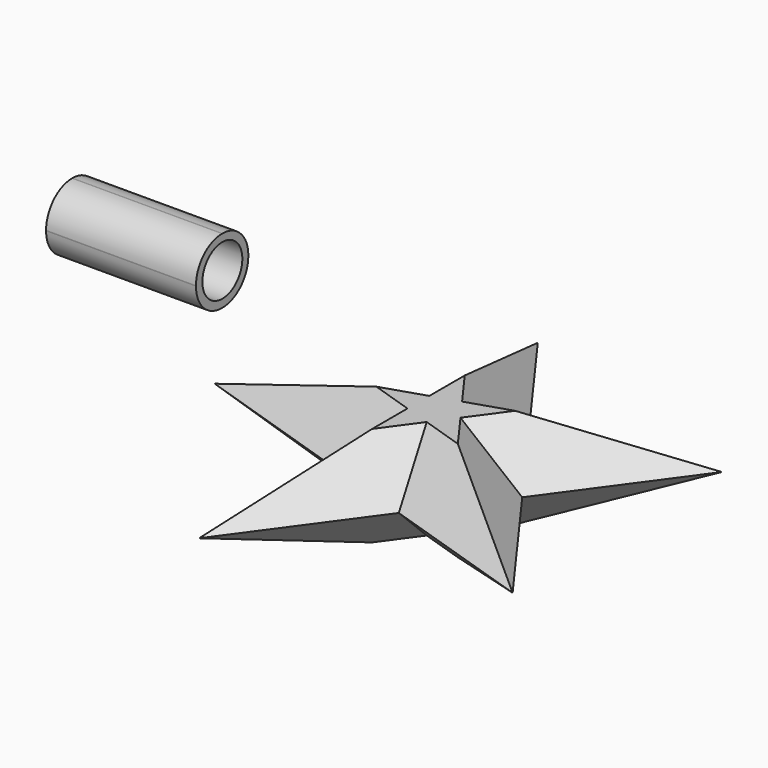
from build123d import *

# Parameters (mm, degrees)
F1_DEPTH      = 25.4
F2_T4_DEPTH   = 106.4188112086
F2_T9_DEPTH   = 106.4188112086
F2_T14_DEPTH  = 106.4188112086
F2_T19_DEPTH  = 106.4188112086
F2_T24_DEPTH  = 106.4188112086
F2_T29_DEPTH  = 106.4188112086
F2_T34_DEPTH  = 106.4188112086
F2_T39_DEPTH  = 106.4188112086
F2_T44_DEPTH  = 106.4188112086
F2_T49_DEPTH  = 106.4188112086
F2_T54_DEPTH  = 106.4188112086
F2_T59_DEPTH  = 106.4188112086
F2_T64_DEPTH  = 106.4188112086
F2_T69_DEPTH  = 106.4188112086
F2_T74_DEPTH  = 106.4188112086
F2_T79_DEPTH  = 106.4188112086
F2_T84_DEPTH  = 106.4188112086
F2_T89_DEPTH  = 106.4188112086
F2_T94_DEPTH  = 106.4188112086
F2_T99_DEPTH  = 106.4188112086
F2_T104_DEPTH = 106.4188112086
F2_T109_DEPTH = 106.4188112086
F2_T114_DEPTH = 106.4188112086
F2_T119_DEPTH = 106.4188112086
F2_T124_DEPTH = 106.4188112086
F2_T129_DEPTH = 106.4188112086
F2_T134_DEPTH = 106.4188112086
F2_T139_DEPTH = 106.4188112086
F2_T144_DEPTH = 106.4188112086
F2_T149_DEPTH = 106.4188112086
F2_T154_DEPTH = 106.4188112086
F2_T159_DEPTH = 106.4188112086
F2_T164_DEPTH = 106.4188112086
F2_T169_DEPTH = 106.4188112086
F2_T174_DEPTH = 106.4188112086
F2_T179_DEPTH = 106.4188112086
F2_T184_DEPTH = 106.4188112086
F2_T189_DEPTH = 106.4188112086
F2_T194_DEPTH = 106.4188112086
F2_T199_DEPTH = 106.4188112086
F2_T205_DEPTH = 106.4188112086
F2_T210_DEPTH = 106.4188112086
F2_T218_DEPTH = 106.4188112086
F2_T223_DEPTH = 106.4188112086
F2_T231_DEPTH = 106.4188112086
F2_T236_DEPTH = 106.4188112086
F2_T244_DEPTH = 106.4188112086
F2_T249_DEPTH = 106.4188112086
F2_T257_DEPTH = 106.4188112086
F2_T262_DEPTH = 106.4188112086
F2_T270_DEPTH = 106.4188112086
F2_T275_DEPTH = 106.4188112086
F2_T283_DEPTH = 106.4188112086
F2_T288_DEPTH = 106.4188112086
F2_T296_DEPTH = 106.4188112086
F2_T301_DEPTH = 106.4188112086
F2_T309_DEPTH = 106.4188112086
F2_T314_DEPTH = 106.4188112086
F2_T322_DEPTH = 106.4188112086
F2_T327_DEPTH = 106.4188112086
F3_W          = 38.1
F3_H          = 16.637
F4_DEPTH      = 16.637
F5_R          = 8.255
F6_R          = 6.35
F7_DEPTH      = 33.02


# Not quite as in the source:
# - a fillet or chamfer that OpenCascade refuses, or shapes differently, is made with other operations: its cross-section is extruded or revolved along the edge and cut away or added


with BuildPart() as f1:
    # F0 (on Top) → F1 (new body)
    with BuildSketch(Plane.XY):
        Polygon((45.763366046, 33.2490316571), (6.6767851239, 20.5490316571), (-17.48005039, 53.7980633142), (-17.48005039, 12.7), (-56.5666313121, 0), (-17.48005039, -12.7), (-17.48005039, -53.7980633142), (-5.401632633, -37.1735474857), (6.6767851239, -20.5490316571), (26.220075585, -26.8990316571), (45.763366046, -33.2490316571), (33.6849482891, -16.6245158286), (27.6457394106, -8.3122579143), (21.6065305321, 0), (27.6457394106, 8.3122579143), (33.6849482891, 16.6245158286), align=None)
    extrude(amount=F1_DEPTH)

    # F2: chamfer of 12.7 on 20 edges, made by hand


with BuildPart() as f2_tool2:
    # F2_s3 → F2_t4 (new body)
    with BuildSketch(Plane(origin=(82.2268601462, 26.7171264209, 0), x_dir=(0, 0, 1), z_dir=(-0.9510565163, -0.3090169944, 0))):
        Polygon((12.7, 17.48005039), (0, 4.78005039), (0, 17.48005039), align=None)
    extrude(amount=F2_T4_DEPTH)

    split(bisect_by=Plane(origin=(14.141657828, 10.2745158286, 0), x_dir=(0, 0, 1), z_dir=(0.8090169944, 0.5877852523, 0)), keep=Keep.TOP)


with BuildPart() as f1_1:
    add(f1.part)

    # F2_t1: cut F2_tool2
    add(f2_tool2.part, mode=Mode.SUBTRACT)


with BuildPart() as f2_tool7:
    # F2_s8 → F2_t9 (new body)
    with BuildSketch(Plane(origin=(82.2268601462, 26.7171264209, 0), x_dir=(0, 0, 1), z_dir=(-0.9510565163, -0.3090169944, 0))):
        Polygon((12.7, 17.48005039), (0, 4.78005039), (0, 17.48005039), align=None)
    extrude(amount=F2_T9_DEPTH)

    split(bisect_by=Plane.YZ.offset(-17.48005039), keep=Keep.BOTTOM)


with BuildPart() as f1_2:
    add(f1_1.part)

    # F2_t6: cut F2_tool7
    add(f2_tool7.part, mode=Mode.SUBTRACT)


with BuildPart() as f2_tool12:
    # F2_s13 → F2_t14 (new body)
    with BuildSketch(Plane(origin=(11.7324134364, -16.1482817373, 0), x_dir=(0, 0, 1), z_dir=(-0.5877852523, 0.8090169944, 0))):
        Polygon((12.7, 17.48005039), (0, 4.78005039), (0, 17.48005039), align=None)
    extrude(amount=F2_T14_DEPTH)

    split(bisect_by=Plane(origin=(14.141657828, -10.2745158286, 0), x_dir=(0, 0, 1), z_dir=(0.8090169944, -0.5877852523, 0)), keep=Keep.TOP)


with BuildPart() as f1_3:
    add(f1_2.part)

    # F2_t11: cut F2_tool12
    add(f2_tool12.part, mode=Mode.SUBTRACT)


with BuildPart() as f2_tool17:
    # F2_s18 → F2_t19 (new body)
    with BuildSketch(Plane(origin=(11.7324134364, -16.1482817373, 0), x_dir=(0, 0, 1), z_dir=(-0.5877852523, 0.8090169944, 0))):
        Polygon((12.7, 17.48005039), (0, 4.78005039), (0, 17.48005039), align=None)
    extrude(amount=F2_T19_DEPTH)

    split(bisect_by=Plane(origin=(-5.401632633, 16.6245158286, 0), x_dir=(0, 0, 1), z_dir=(-0.3090169944, 0.9510565163, 0)), keep=Keep.TOP)


with BuildPart() as f1_4:
    add(f1_3.part)

    # F2_t16: cut F2_tool17
    add(f2_tool17.part, mode=Mode.SUBTRACT)


with BuildPart() as f2_tool22:
    # F2_s23 → F2_t24 (new body)
    with BuildSketch(Plane.XZ.offset(-86.4584372614)):
        Polygon((-17.48005039, 12.7), (-4.78005039, 0), (-17.48005039, 0), align=None)
    extrude(amount=F2_T24_DEPTH)

    split(bisect_by=Plane(origin=(-5.401632633, 16.6245158286, 0), x_dir=(0, 0, 1), z_dir=(-0.3090169944, 0.9510565163, 0)), keep=Keep.TOP)


with BuildPart() as f1_5:
    add(f1_4.part)

    # F2_t21: cut F2_tool22
    add(f2_tool22.part, mode=Mode.SUBTRACT)


with BuildPart() as f2_tool27:
    # F2_s28 → F2_t29 (new body)
    with BuildSketch(Plane.XZ.offset(-86.4584372614)):
        Polygon((-17.48005039, 12.7), (-4.78005039, 0), (-17.48005039, 0), align=None)
    extrude(amount=F2_T29_DEPTH)

    split(bisect_by=Plane(origin=(-5.401632633, -16.6245158286, 0), x_dir=(0, 0, 1), z_dir=(-0.3090169944, -0.9510565163, 0)), keep=Keep.TOP)


with BuildPart() as f1_6:
    add(f1_5.part)

    # F2_t26: cut F2_tool27
    add(f2_tool27.part, mode=Mode.SUBTRACT)


with BuildPart() as f2_tool32:
    # F2_s33 → F2_t34 (new body)
    with BuildSketch(Plane(origin=(18.9834437101, 6.1680947638, 0), x_dir=(0, 0, 1), z_dir=(-0.9510565163, -0.3090169944, 0))):
        Polygon((12.7, 17.48005039), (0, 4.78005039), (0, 17.48005039), align=None)
    extrude(amount=F2_T34_DEPTH)

    split(bisect_by=Plane(origin=(14.141657828, 10.2745158286, 0), x_dir=(0, 0, 1), z_dir=(0.8090169944, 0.5877852523, 0)), keep=Keep.TOP)


with BuildPart() as f1_7:
    add(f1_6.part)

    # F2_t31: cut F2_tool32
    add(f2_tool32.part, mode=Mode.SUBTRACT)


with BuildPart() as f2_tool37:
    # F2_s38 → F2_t39 (new body)
    with BuildSketch(Plane(origin=(18.9834437101, 6.1680947638, 0), x_dir=(0, 0, 1), z_dir=(-0.9510565163, -0.3090169944, 0))):
        Polygon((12.7, 17.48005039), (0, 4.78005039), (0, 17.48005039), align=None)
    extrude(amount=F2_T39_DEPTH)

    split(bisect_by=Plane.YZ.offset(-17.48005039), keep=Keep.BOTTOM)


with BuildPart() as f1_8:
    add(f1_7.part)

    # F2_t36: cut F2_tool37
    add(f2_tool37.part, mode=Mode.SUBTRACT)


with BuildPart() as f2_tool42:
    # F2_s43 → F2_t44 (new body)
    with BuildSketch(Plane(origin=(-82.2268601462, 26.7171264209, 0), x_dir=(0, 0, 1), z_dir=(0.9510565163, -0.3090169944, 0))):
        Polygon((12.7, 17.48005039), (0, 4.78005039), (0, 17.48005039), align=None)
    extrude(amount=F2_T44_DEPTH)

    split(bisect_by=Plane.YZ.offset(-17.48005039), keep=Keep.BOTTOM)


with BuildPart() as f1_9:
    add(f1_8.part)

    # F2_t41: cut F2_tool42
    add(f2_tool42.part, mode=Mode.SUBTRACT)


with BuildPart() as f2_tool47:
    # F2_s48 → F2_t49 (new body)
    with BuildSketch(Plane(origin=(-82.2268601462, 26.7171264209, 0), x_dir=(0, 0, 1), z_dir=(0.9510565163, -0.3090169944, 0))):
        Polygon((12.7, 17.48005039), (0, 4.78005039), (0, 17.48005039), align=None)
    extrude(amount=F2_T49_DEPTH)

    split(bisect_by=Plane(origin=(14.141657828, -10.2745158286, 0), x_dir=(0, 0, 1), z_dir=(0.8090169944, -0.5877852523, 0)), keep=Keep.TOP)


with BuildPart() as f1_10:
    add(f1_9.part)

    # F2_t46: cut F2_tool47
    add(f2_tool47.part, mode=Mode.SUBTRACT)


with BuildPart() as f2_tool52:
    # F2_s53 → F2_t54 (new body)
    with BuildSketch(Plane.XZ.offset(-19.9603739472)):
        Polygon((-17.48005039, 12.7), (-4.78005039, 0), (-17.48005039, 0), align=None)
    extrude(amount=F2_T54_DEPTH)

    split(bisect_by=Plane(origin=(-5.401632633, 16.6245158286, 0), x_dir=(0, 0, 1), z_dir=(-0.3090169944, 0.9510565163, 0)), keep=Keep.TOP)


with BuildPart() as f1_11:
    add(f1_10.part)

    # F2_t51: cut F2_tool52
    add(f2_tool52.part, mode=Mode.SUBTRACT)


with BuildPart() as f2_tool57:
    # F2_s58 → F2_t59 (new body)
    with BuildSketch(Plane.XZ.offset(-19.9603739472)):
        Polygon((-17.48005039, 12.7), (-4.78005039, 0), (-17.48005039, 0), align=None)
    extrude(amount=F2_T59_DEPTH)

    split(bisect_by=Plane(origin=(-5.401632633, -16.6245158286, 0), x_dir=(0, 0, 1), z_dir=(-0.3090169944, -0.9510565163, 0)), keep=Keep.TOP)


with BuildPart() as f1_12:
    add(f1_11.part)

    # F2_t56: cut F2_tool57
    add(f2_tool57.part, mode=Mode.SUBTRACT)


with BuildPart() as f2_tool62:
    # F2_s63 → F2_t64 (new body)
    with BuildSketch(Plane(origin=(-50.8189943585, -69.9463450516, 0), x_dir=(0, 0, 1), z_dir=(0.5877852523, 0.8090169944, 0))):
        Polygon((12.7, 17.48005039), (0, 4.78005039), (0, 17.48005039), align=None)
    extrude(amount=F2_T64_DEPTH)

    split(bisect_by=Plane(origin=(-5.401632633, -16.6245158286, 0), x_dir=(0, 0, 1), z_dir=(-0.3090169944, -0.9510565163, 0)), keep=Keep.TOP)


with BuildPart() as f1_13:
    add(f1_12.part)

    # F2_t61: cut F2_tool62
    add(f2_tool62.part, mode=Mode.SUBTRACT)


with BuildPart() as f2_tool67:
    # F2_s68 → F2_t69 (new body)
    with BuildSketch(Plane(origin=(-50.8189943585, -69.9463450516, 0), x_dir=(0, 0, 1), z_dir=(0.5877852523, 0.8090169944, 0))):
        Polygon((12.7, 17.48005039), (0, 4.78005039), (0, 17.48005039), align=None)
    extrude(amount=F2_T69_DEPTH)

    split(bisect_by=Plane(origin=(14.141657828, 10.2745158286, 0), x_dir=(0, 0, 1), z_dir=(0.8090169944, 0.5877852523, 0)), keep=Keep.TOP)


with BuildPart() as f1_14:
    add(f1_13.part)

    # F2_t66: cut F2_tool67
    add(f2_tool67.part, mode=Mode.SUBTRACT)


with BuildPart() as f2_tool72:
    # F2_s73 → F2_t74 (new body)
    with BuildSketch(Plane(origin=(-18.9834437101, 6.1680947638, 0), x_dir=(0, 0, 1), z_dir=(0.9510565163, -0.3090169944, 0))):
        Polygon((12.7, 17.48005039), (0, 4.78005039), (0, 17.48005039), align=None)
    extrude(amount=F2_T74_DEPTH)

    split(bisect_by=Plane.YZ.offset(-17.48005039), keep=Keep.BOTTOM)


with BuildPart() as f1_15:
    add(f1_14.part)

    # F2_t71: cut F2_tool72
    add(f2_tool72.part, mode=Mode.SUBTRACT)


with BuildPart() as f2_tool77:
    # F2_s78 → F2_t79 (new body)
    with BuildSketch(Plane(origin=(-18.9834437101, 6.1680947638, 0), x_dir=(0, 0, 1), z_dir=(0.9510565163, -0.3090169944, 0))):
        Polygon((12.7, 17.48005039), (0, 4.78005039), (0, 17.48005039), align=None)
    extrude(amount=F2_T79_DEPTH)

    split(bisect_by=Plane(origin=(14.141657828, -10.2745158286, 0), x_dir=(0, 0, 1), z_dir=(0.8090169944, -0.5877852523, 0)), keep=Keep.TOP)


with BuildPart() as f1_16:
    add(f1_15.part)

    # F2_t76: cut F2_tool77
    add(f2_tool77.part, mode=Mode.SUBTRACT)


with BuildPart() as f2_tool82:
    # F2_s83 → F2_t84 (new body)
    with BuildSketch(Plane(origin=(50.8189943585, -69.9463450516, 0), x_dir=(0, 0, 1), z_dir=(-0.5877852523, 0.8090169944, 0))):
        Polygon((12.7, 17.48005039), (0, 4.78005039), (0, 17.48005039), align=None)
    extrude(amount=F2_T84_DEPTH)

    split(bisect_by=Plane(origin=(14.141657828, -10.2745158286, 0), x_dir=(0, 0, 1), z_dir=(0.8090169944, -0.5877852523, 0)), keep=Keep.TOP)


with BuildPart() as f1_17:
    add(f1_16.part)

    # F2_t81: cut F2_tool82
    add(f2_tool82.part, mode=Mode.SUBTRACT)


with BuildPart() as f2_tool87:
    # F2_s88 → F2_t89 (new body)
    with BuildSketch(Plane(origin=(50.8189943585, -69.9463450516, 0), x_dir=(0, 0, 1), z_dir=(-0.5877852523, 0.8090169944, 0))):
        Polygon((12.7, 17.48005039), (0, 4.78005039), (0, 17.48005039), align=None)
    extrude(amount=F2_T89_DEPTH)

    split(bisect_by=Plane(origin=(-5.401632633, 16.6245158286, 0), x_dir=(0, 0, 1), z_dir=(-0.3090169944, 0.9510565163, 0)), keep=Keep.TOP)


with BuildPart() as f1_18:
    add(f1_17.part)

    # F2_t86: cut F2_tool87
    add(f2_tool87.part, mode=Mode.SUBTRACT)


with BuildPart() as f2_tool92:
    # F2_s93 → F2_t94 (new body)
    with BuildSketch(Plane(origin=(-11.7324134364, -16.1482817373, 0), x_dir=(0, 0, 1), z_dir=(0.5877852523, 0.8090169944, 0))):
        Polygon((12.7, 17.48005039), (0, 4.78005039), (0, 17.48005039), align=None)
    extrude(amount=F2_T94_DEPTH)

    split(bisect_by=Plane(origin=(-5.401632633, -16.6245158286, 0), x_dir=(0, 0, 1), z_dir=(-0.3090169944, -0.9510565163, 0)), keep=Keep.TOP)


with BuildPart() as f1_19:
    add(f1_18.part)

    # F2_t91: cut F2_tool92
    add(f2_tool92.part, mode=Mode.SUBTRACT)


with BuildPart() as f2_tool97:
    # F2_s98 → F2_t99 (new body)
    with BuildSketch(Plane(origin=(-11.7324134364, -16.1482817373, 0), x_dir=(0, 0, 1), z_dir=(0.5877852523, 0.8090169944, 0))):
        Polygon((12.7, 17.48005039), (0, 4.78005039), (0, 17.48005039), align=None)
    extrude(amount=F2_T99_DEPTH)

    split(bisect_by=Plane(origin=(14.141657828, 10.2745158286, 0), x_dir=(0, 0, 1), z_dir=(0.8090169944, 0.5877852523, 0)), keep=Keep.TOP)


with BuildPart() as f1_20:
    add(f1_19.part)

    # F2_t96: cut F2_tool97
    add(f2_tool97.part, mode=Mode.SUBTRACT)


with BuildPart() as f2_tool102:
    # F2_s103 → F2_t104 (new body)
    with BuildSketch(Plane(origin=(50.8189943585, 69.9463450516, 0), x_dir=(0, 0, 1), z_dir=(-0.5877852523, -0.8090169944, 0))):
        Polygon((12.7, -17.48005039), (25.4, -4.78005039), (25.4, -17.48005039), align=None)
    extrude(amount=F2_T104_DEPTH)

    split(bisect_by=Plane(origin=(14.141657828, 10.2745158286, 0), x_dir=(0, 0, 1), z_dir=(0.8090169944, 0.5877852523, 0)), keep=Keep.TOP)


with BuildPart() as f1_21:
    add(f1_20.part)

    # F2_t101: cut F2_tool102
    add(f2_tool102.part, mode=Mode.SUBTRACT)


with BuildPart() as f2_tool107:
    # F2_s108 → F2_t109 (new body)
    with BuildSketch(Plane(origin=(50.8189943585, 69.9463450516, 0), x_dir=(0, 0, 1), z_dir=(-0.5877852523, -0.8090169944, 0))):
        Polygon((12.7, -17.48005039), (25.4, -4.78005039), (25.4, -17.48005039), align=None)
    extrude(amount=F2_T109_DEPTH)

    split(bisect_by=Plane(origin=(-5.401632633, -16.6245158286, 0), x_dir=(0, 0, 1), z_dir=(-0.3090169944, -0.9510565163, 0)), keep=Keep.TOP)


with BuildPart() as f1_22:
    add(f1_21.part)

    # F2_t106: cut F2_tool107
    add(f2_tool107.part, mode=Mode.SUBTRACT)


with BuildPart() as f2_tool112:
    # F2_s113 → F2_t114 (new body)
    with BuildSketch(Plane(origin=(82.2268601462, 26.7171264209, 0), x_dir=(0, 0, 1), z_dir=(-0.9510565163, -0.3090169944, 0))):
        Polygon((12.7, 17.48005039), (25.4, 4.78005039), (25.4, 17.48005039), align=None)
    extrude(amount=F2_T114_DEPTH)

    split(bisect_by=Plane(origin=(14.141657828, 10.2745158286, 0), x_dir=(0, 0, 1), z_dir=(0.8090169944, 0.5877852523, 0)), keep=Keep.TOP)


with BuildPart() as f1_23:
    add(f1_22.part)

    # F2_t111: cut F2_tool112
    add(f2_tool112.part, mode=Mode.SUBTRACT)


with BuildPart() as f2_tool117:
    # F2_s118 → F2_t119 (new body)
    with BuildSketch(Plane(origin=(82.2268601462, 26.7171264209, 0), x_dir=(0, 0, 1), z_dir=(-0.9510565163, -0.3090169944, 0))):
        Polygon((12.7, 17.48005039), (25.4, 4.78005039), (25.4, 17.48005039), align=None)
    extrude(amount=F2_T119_DEPTH)

    split(bisect_by=Plane.YZ.offset(-17.48005039), keep=Keep.BOTTOM)


with BuildPart() as f1_24:
    add(f1_23.part)

    # F2_t116: cut F2_tool117
    add(f2_tool117.part, mode=Mode.SUBTRACT)


with BuildPart() as f2_tool122:
    # F2_s123 → F2_t124 (new body)
    with BuildSketch(Plane(origin=(11.7324134364, -16.1482817373, 0), x_dir=(0, 0, 1), z_dir=(-0.5877852523, 0.8090169944, 0))):
        Polygon((12.7, 17.48005039), (25.4, 4.78005039), (25.4, 17.48005039), align=None)
    extrude(amount=F2_T124_DEPTH)

    split(bisect_by=Plane(origin=(14.141657828, -10.2745158286, 0), x_dir=(0, 0, 1), z_dir=(0.8090169944, -0.5877852523, 0)), keep=Keep.TOP)


with BuildPart() as f1_25:
    add(f1_24.part)

    # F2_t121: cut F2_tool122
    add(f2_tool122.part, mode=Mode.SUBTRACT)


with BuildPart() as f2_tool127:
    # F2_s128 → F2_t129 (new body)
    with BuildSketch(Plane(origin=(11.7324134364, -16.1482817373, 0), x_dir=(0, 0, 1), z_dir=(-0.5877852523, 0.8090169944, 0))):
        Polygon((12.7, 17.48005039), (25.4, 4.78005039), (25.4, 17.48005039), align=None)
    extrude(amount=F2_T129_DEPTH)

    split(bisect_by=Plane(origin=(-5.401632633, 16.6245158286, 0), x_dir=(0, 0, 1), z_dir=(-0.3090169944, 0.9510565163, 0)), keep=Keep.TOP)


with BuildPart() as f1_26:
    add(f1_25.part)

    # F2_t126: cut F2_tool127
    add(f2_tool127.part, mode=Mode.SUBTRACT)


with BuildPart() as f2_tool132:
    # F2_s133 → F2_t134 (new body)
    with BuildSketch(Plane.XZ.offset(-86.4584372614)):
        Polygon((-17.48005039, 12.7), (-4.78005039, 25.4), (-17.48005039, 25.4), align=None)
    extrude(amount=F2_T134_DEPTH)

    split(bisect_by=Plane(origin=(-5.401632633, 16.6245158286, 0), x_dir=(0, 0, 1), z_dir=(-0.3090169944, 0.9510565163, 0)), keep=Keep.TOP)


with BuildPart() as f1_27:
    add(f1_26.part)

    # F2_t131: cut F2_tool132
    add(f2_tool132.part, mode=Mode.SUBTRACT)


with BuildPart() as f2_tool137:
    # F2_s138 → F2_t139 (new body)
    with BuildSketch(Plane.XZ.offset(-86.4584372614)):
        Polygon((-17.48005039, 12.7), (-4.78005039, 25.4), (-17.48005039, 25.4), align=None)
    extrude(amount=F2_T139_DEPTH)

    split(bisect_by=Plane(origin=(-5.401632633, -16.6245158286, 0), x_dir=(0, 0, 1), z_dir=(-0.3090169944, -0.9510565163, 0)), keep=Keep.TOP)


with BuildPart() as f1_28:
    add(f1_27.part)

    # F2_t136: cut F2_tool137
    add(f2_tool137.part, mode=Mode.SUBTRACT)


with BuildPart() as f2_tool142:
    # F2_s143 → F2_t144 (new body)
    with BuildSketch(Plane(origin=(18.9834437101, 6.1680947638, 0), x_dir=(0, 0, 1), z_dir=(-0.9510565163, -0.3090169944, 0))):
        Polygon((12.7, 17.48005039), (25.4, 4.78005039), (25.4, 17.48005039), align=None)
    extrude(amount=F2_T144_DEPTH)

    split(bisect_by=Plane(origin=(14.141657828, 10.2745158286, 0), x_dir=(0, 0, 1), z_dir=(0.8090169944, 0.5877852523, 0)), keep=Keep.TOP)


with BuildPart() as f1_29:
    add(f1_28.part)

    # F2_t141: cut F2_tool142
    add(f2_tool142.part, mode=Mode.SUBTRACT)


with BuildPart() as f2_tool147:
    # F2_s148 → F2_t149 (new body)
    with BuildSketch(Plane(origin=(18.9834437101, 6.1680947638, 0), x_dir=(0, 0, 1), z_dir=(-0.9510565163, -0.3090169944, 0))):
        Polygon((12.7, 17.48005039), (25.4, 4.78005039), (25.4, 17.48005039), align=None)
    extrude(amount=F2_T149_DEPTH)

    split(bisect_by=Plane.YZ.offset(-17.48005039), keep=Keep.BOTTOM)


with BuildPart() as f1_30:
    add(f1_29.part)

    # F2_t146: cut F2_tool147
    add(f2_tool147.part, mode=Mode.SUBTRACT)


with BuildPart() as f2_tool152:
    # F2_s153 → F2_t154 (new body)
    with BuildSketch(Plane(origin=(-82.2268601462, 26.7171264209, 0), x_dir=(0, 0, 1), z_dir=(0.9510565163, -0.3090169944, 0))):
        Polygon((12.7, 17.48005039), (25.4, 4.78005039), (25.4, 17.48005039), align=None)
    extrude(amount=F2_T154_DEPTH)

    split(bisect_by=Plane.YZ.offset(-17.48005039), keep=Keep.BOTTOM)


with BuildPart() as f1_31:
    add(f1_30.part)

    # F2_t151: cut F2_tool152
    add(f2_tool152.part, mode=Mode.SUBTRACT)


with BuildPart() as f2_tool157:
    # F2_s158 → F2_t159 (new body)
    with BuildSketch(Plane(origin=(-82.2268601462, 26.7171264209, 0), x_dir=(0, 0, 1), z_dir=(0.9510565163, -0.3090169944, 0))):
        Polygon((12.7, 17.48005039), (25.4, 4.78005039), (25.4, 17.48005039), align=None)
    extrude(amount=F2_T159_DEPTH)

    split(bisect_by=Plane(origin=(14.141657828, -10.2745158286, 0), x_dir=(0, 0, 1), z_dir=(0.8090169944, -0.5877852523, 0)), keep=Keep.TOP)


with BuildPart() as f1_32:
    add(f1_31.part)

    # F2_t156: cut F2_tool157
    add(f2_tool157.part, mode=Mode.SUBTRACT)


with BuildPart() as f2_tool162:
    # F2_s163 → F2_t164 (new body)
    with BuildSketch(Plane.XZ.offset(-19.9603739472)):
        Polygon((-17.48005039, 12.7), (-4.78005039, 25.4), (-17.48005039, 25.4), align=None)
    extrude(amount=F2_T164_DEPTH)

    split(bisect_by=Plane(origin=(-5.401632633, 16.6245158286, 0), x_dir=(0, 0, 1), z_dir=(-0.3090169944, 0.9510565163, 0)), keep=Keep.TOP)


with BuildPart() as f1_33:
    add(f1_32.part)

    # F2_t161: cut F2_tool162
    add(f2_tool162.part, mode=Mode.SUBTRACT)


with BuildPart() as f2_tool167:
    # F2_s168 → F2_t169 (new body)
    with BuildSketch(Plane.XZ.offset(-19.9603739472)):
        Polygon((-17.48005039, 12.7), (-4.78005039, 25.4), (-17.48005039, 25.4), align=None)
    extrude(amount=F2_T169_DEPTH)

    split(bisect_by=Plane(origin=(-5.401632633, -16.6245158286, 0), x_dir=(0, 0, 1), z_dir=(-0.3090169944, -0.9510565163, 0)), keep=Keep.TOP)


with BuildPart() as f1_34:
    add(f1_33.part)

    # F2_t166: cut F2_tool167
    add(f2_tool167.part, mode=Mode.SUBTRACT)


with BuildPart() as f2_tool172:
    # F2_s173 → F2_t174 (new body)
    with BuildSketch(Plane(origin=(11.7324134364, 16.1482817373, 0), x_dir=(0, 0, 1), z_dir=(-0.5877852523, -0.8090169944, 0))):
        Polygon((12.7, -17.48005039), (25.4, -4.78005039), (25.4, -17.48005039), align=None)
    extrude(amount=F2_T174_DEPTH)

    split(bisect_by=Plane(origin=(14.141657828, 10.2745158286, 0), x_dir=(0, 0, 1), z_dir=(0.8090169944, 0.5877852523, 0)), keep=Keep.TOP)


with BuildPart() as f1_35:
    add(f1_34.part)

    # F2_t171: cut F2_tool172
    add(f2_tool172.part, mode=Mode.SUBTRACT)


with BuildPart() as f2_tool177:
    # F2_s178 → F2_t179 (new body)
    with BuildSketch(Plane(origin=(11.7324134364, 16.1482817373, 0), x_dir=(0, 0, 1), z_dir=(-0.5877852523, -0.8090169944, 0))):
        Polygon((12.7, -17.48005039), (25.4, -4.78005039), (25.4, -17.48005039), align=None)
    extrude(amount=F2_T179_DEPTH)

    split(bisect_by=Plane(origin=(-5.401632633, -16.6245158286, 0), x_dir=(0, 0, 1), z_dir=(-0.3090169944, -0.9510565163, 0)), keep=Keep.TOP)


with BuildPart() as f1_36:
    add(f1_35.part)

    # F2_t176: cut F2_tool177
    add(f2_tool177.part, mode=Mode.SUBTRACT)


with BuildPart() as f2_tool182:
    # F2_s183 → F2_t184 (new body)
    with BuildSketch(Plane(origin=(82.2268601462, -26.7171264209, 0), x_dir=(0, 0, 1), z_dir=(-0.9510565163, 0.3090169944, 0))):
        Polygon((12.7, -17.48005039), (25.4, -4.78005039), (25.4, -17.48005039), align=None)
    extrude(amount=F2_T184_DEPTH)

    split(bisect_by=Plane(origin=(14.141657828, -10.2745158286, 0), x_dir=(0, 0, 1), z_dir=(0.8090169944, -0.5877852523, 0)), keep=Keep.TOP)


with BuildPart() as f1_37:
    add(f1_36.part)

    # F2_t181: cut F2_tool182
    add(f2_tool182.part, mode=Mode.SUBTRACT)


with BuildPart() as f2_tool187:
    # F2_s188 → F2_t189 (new body)
    with BuildSketch(Plane(origin=(82.2268601462, -26.7171264209, 0), x_dir=(0, 0, 1), z_dir=(-0.9510565163, 0.3090169944, 0))):
        Polygon((12.7, -17.48005039), (25.4, -4.78005039), (25.4, -17.48005039), align=None)
    extrude(amount=F2_T189_DEPTH)

    split(bisect_by=Plane.YZ.offset(-17.48005039), keep=Keep.BOTTOM)


with BuildPart() as f1_38:
    add(f1_37.part)

    # F2_t186: cut F2_tool187
    add(f2_tool187.part, mode=Mode.SUBTRACT)


with BuildPart() as f2_tool192:
    # F2_s193 → F2_t194 (new body)
    with BuildSketch(Plane(origin=(-11.7324134364, 16.1482817373, 0), x_dir=(0, 0, 1), z_dir=(0.5877852523, -0.8090169944, 0))):
        Polygon((25.4, -4.78005039), (12.7, -17.48005039), (25.4, -17.48005039), align=None)
    extrude(amount=F2_T194_DEPTH)

    split(bisect_by=Plane(origin=(-5.401632633, 16.6245158286, 0), x_dir=(0, 0, 1), z_dir=(-0.3090169944, 0.9510565163, 0)), keep=Keep.TOP)


with BuildPart() as f1_39:
    add(f1_38.part)

    # F2_t191: cut F2_tool192
    add(f2_tool192.part, mode=Mode.SUBTRACT)


with BuildPart() as f2_tool197:
    # F2_s198 → F2_t199 (new body)
    with BuildSketch(Plane(origin=(-11.7324134364, 16.1482817373, 0), x_dir=(0, 0, 1), z_dir=(0.5877852523, -0.8090169944, 0))):
        Polygon((25.4, -4.78005039), (12.7, -17.48005039), (25.4, -17.48005039), align=None)
    extrude(amount=F2_T199_DEPTH)

    split(bisect_by=Plane(origin=(14.141657828, -10.2745158286, 0), x_dir=(0, 0, 1), z_dir=(0.8090169944, -0.5877852523, 0)), keep=Keep.TOP)


with BuildPart() as f1_40:
    add(f1_39.part)

    # F2_t196: cut F2_tool197
    add(f2_tool197.part, mode=Mode.SUBTRACT)


with BuildPart() as f2_tool203:
    # F2_s204 → F2_t205 (new body)
    with BuildSketch(Plane(origin=(82.2268601462, 26.7171264209, 0), x_dir=(0, 0, 1), z_dir=(-0.9510565163, -0.3090169944, 0))):
        Polygon((12.7, 17.48005039), (0, 4.78005039), (0, 17.48005039), align=None)
    extrude(amount=F2_T205_DEPTH)

    split(bisect_by=Plane(origin=(14.141657828, 10.2745158286, 0), x_dir=(0, 0, 1), z_dir=(-0.8090169944, -0.5877852523, 0)), keep=Keep.TOP)

    split(bisect_by=Plane.YZ.offset(-17.48005039), keep=Keep.TOP)


with BuildPart() as f2_tool208:
    # F2_s209 → F2_t210 (new body)
    with BuildSketch(Plane(origin=(11.7324134364, -16.1482817373, 0), x_dir=(0, 0, 1), z_dir=(-0.5877852523, 0.8090169944, 0))):
        Polygon((12.7, 17.48005039), (0, 4.78005039), (0, 17.48005039), align=None)
    extrude(amount=F2_T210_DEPTH)

    split(bisect_by=Plane(origin=(14.141657828, -10.2745158286, 0), x_dir=(0, 0, 1), z_dir=(-0.8090169944, 0.5877852523, 0)), keep=Keep.TOP)

    split(bisect_by=Plane(origin=(-5.401632633, 16.6245158286, 0), x_dir=(0, 0, 1), z_dir=(0.3090169944, -0.9510565163, 0)), keep=Keep.TOP)


with BuildPart() as f2_tool203_1:
    add(f2_tool203.part)

    # F2_t213: intersect F2_tool208
    add(f2_tool208.part, mode=Mode.INTERSECT)


with BuildPart() as f1_41:
    add(f1_40.part)

    # F2_t201: cut F2_tool203
    add(f2_tool203_1.part, mode=Mode.SUBTRACT)


with BuildPart() as f2_tool216:
    # F2_s217 → F2_t218 (new body)
    with BuildSketch(Plane.XZ.offset(-86.4584372614)):
        Polygon((-17.48005039, 12.7), (-4.78005039, 0), (-17.48005039, 0), align=None)
    extrude(amount=F2_T218_DEPTH)

    split(bisect_by=Plane(origin=(-5.401632633, 16.6245158286, 0), x_dir=(0, 0, 1), z_dir=(0.3090169944, -0.9510565163, 0)), keep=Keep.TOP)

    split(bisect_by=Plane(origin=(-5.401632633, -16.6245158286, 0), x_dir=(0, 0, 1), z_dir=(0.3090169944, 0.9510565163, 0)), keep=Keep.TOP)


with BuildPart() as f2_tool221:
    # F2_s222 → F2_t223 (new body)
    with BuildSketch(Plane(origin=(18.9834437101, 6.1680947638, 0), x_dir=(0, 0, 1), z_dir=(-0.9510565163, -0.3090169944, 0))):
        Polygon((12.7, 17.48005039), (0, 4.78005039), (0, 17.48005039), align=None)
    extrude(amount=F2_T223_DEPTH)

    split(bisect_by=Plane(origin=(14.141657828, 10.2745158286, 0), x_dir=(0, 0, 1), z_dir=(-0.8090169944, -0.5877852523, 0)), keep=Keep.TOP)

    split(bisect_by=Plane.YZ.offset(-17.48005039), keep=Keep.TOP)


with BuildPart() as f2_tool216_1:
    add(f2_tool216.part)

    # F2_t226: intersect F2_tool221
    add(f2_tool221.part, mode=Mode.INTERSECT)


with BuildPart() as f1_42:
    add(f1_41.part)

    # F2_t214: cut F2_tool216
    add(f2_tool216_1.part, mode=Mode.SUBTRACT)


with BuildPart() as f2_tool229:
    # F2_s230 → F2_t231 (new body)
    with BuildSketch(Plane(origin=(-82.2268601462, 26.7171264209, 0), x_dir=(0, 0, 1), z_dir=(0.9510565163, -0.3090169944, 0))):
        Polygon((12.7, 17.48005039), (0, 4.78005039), (0, 17.48005039), align=None)
    extrude(amount=F2_T231_DEPTH)

    split(bisect_by=Plane.YZ.offset(-17.48005039), keep=Keep.TOP)

    split(bisect_by=Plane(origin=(14.141657828, -10.2745158286, 0), x_dir=(0, 0, 1), z_dir=(-0.8090169944, 0.5877852523, 0)), keep=Keep.TOP)


with BuildPart() as f2_tool234:
    # F2_s235 → F2_t236 (new body)
    with BuildSketch(Plane.XZ.offset(-19.9603739472)):
        Polygon((-17.48005039, 12.7), (-4.78005039, 0), (-17.48005039, 0), align=None)
    extrude(amount=F2_T236_DEPTH)

    split(bisect_by=Plane(origin=(-5.401632633, 16.6245158286, 0), x_dir=(0, 0, 1), z_dir=(0.3090169944, -0.9510565163, 0)), keep=Keep.TOP)

    split(bisect_by=Plane(origin=(-5.401632633, -16.6245158286, 0), x_dir=(0, 0, 1), z_dir=(0.3090169944, 0.9510565163, 0)), keep=Keep.TOP)


with BuildPart() as f2_tool229_1:
    add(f2_tool229.part)

    # F2_t239: intersect F2_tool234
    add(f2_tool234.part, mode=Mode.INTERSECT)


with BuildPart() as f1_43:
    add(f1_42.part)

    # F2_t227: cut F2_tool229
    add(f2_tool229_1.part, mode=Mode.SUBTRACT)


with BuildPart() as f2_tool242:
    # F2_s243 → F2_t244 (new body)
    with BuildSketch(Plane(origin=(-50.8189943585, -69.9463450516, 0), x_dir=(0, 0, 1), z_dir=(0.5877852523, 0.8090169944, 0))):
        Polygon((12.7, 17.48005039), (0, 4.78005039), (0, 17.48005039), align=None)
    extrude(amount=F2_T244_DEPTH)

    split(bisect_by=Plane(origin=(14.141657828, 10.2745158286, 0), x_dir=(0, 0, 1), z_dir=(-0.8090169944, -0.5877852523, 0)), keep=Keep.TOP)

    split(bisect_by=Plane(origin=(-5.401632633, -16.6245158286, 0), x_dir=(0, 0, 1), z_dir=(0.3090169944, 0.9510565163, 0)), keep=Keep.TOP)


with BuildPart() as f2_tool247:
    # F2_s248 → F2_t249 (new body)
    with BuildSketch(Plane(origin=(-18.9834437101, 6.1680947638, 0), x_dir=(0, 0, 1), z_dir=(0.9510565163, -0.3090169944, 0))):
        Polygon((12.7, 17.48005039), (0, 4.78005039), (0, 17.48005039), align=None)
    extrude(amount=F2_T249_DEPTH)

    split(bisect_by=Plane.YZ.offset(-17.48005039), keep=Keep.TOP)

    split(bisect_by=Plane(origin=(14.141657828, -10.2745158286, 0), x_dir=(0, 0, 1), z_dir=(-0.8090169944, 0.5877852523, 0)), keep=Keep.TOP)


with BuildPart() as f2_tool242_1:
    add(f2_tool242.part)

    # F2_t252: intersect F2_tool247
    add(f2_tool247.part, mode=Mode.INTERSECT)


with BuildPart() as f1_44:
    add(f1_43.part)

    # F2_t240: cut F2_tool242
    add(f2_tool242_1.part, mode=Mode.SUBTRACT)


with BuildPart() as f2_tool255:
    # F2_s256 → F2_t257 (new body)
    with BuildSketch(Plane(origin=(-11.7324134364, -16.1482817373, 0), x_dir=(0, 0, 1), z_dir=(0.5877852523, 0.8090169944, 0))):
        Polygon((12.7, 17.48005039), (0, 4.78005039), (0, 17.48005039), align=None)
    extrude(amount=F2_T257_DEPTH)

    split(bisect_by=Plane(origin=(14.141657828, 10.2745158286, 0), x_dir=(0, 0, 1), z_dir=(-0.8090169944, -0.5877852523, 0)), keep=Keep.TOP)

    split(bisect_by=Plane(origin=(-5.401632633, -16.6245158286, 0), x_dir=(0, 0, 1), z_dir=(0.3090169944, 0.9510565163, 0)), keep=Keep.TOP)


with BuildPart() as f2_tool260:
    # F2_s261 → F2_t262 (new body)
    with BuildSketch(Plane(origin=(50.8189943585, -69.9463450516, 0), x_dir=(0, 0, 1), z_dir=(-0.5877852523, 0.8090169944, 0))):
        Polygon((12.7, 17.48005039), (0, 4.78005039), (0, 17.48005039), align=None)
    extrude(amount=F2_T262_DEPTH)

    split(bisect_by=Plane(origin=(14.141657828, -10.2745158286, 0), x_dir=(0, 0, 1), z_dir=(-0.8090169944, 0.5877852523, 0)), keep=Keep.TOP)

    split(bisect_by=Plane(origin=(-5.401632633, 16.6245158286, 0), x_dir=(0, 0, 1), z_dir=(0.3090169944, -0.9510565163, 0)), keep=Keep.TOP)


with BuildPart() as f2_tool255_1:
    add(f2_tool255.part)

    # F2_t265: intersect F2_tool260
    add(f2_tool260.part, mode=Mode.INTERSECT)


with BuildPart() as f1_45:
    add(f1_44.part)

    # F2_t253: cut F2_tool255
    add(f2_tool255_1.part, mode=Mode.SUBTRACT)


with BuildPart() as f2_tool268:
    # F2_s269 → F2_t270 (new body)
    with BuildSketch(Plane(origin=(50.8189943585, 69.9463450516, 0), x_dir=(0, 0, 1), z_dir=(-0.5877852523, -0.8090169944, 0))):
        Polygon((12.7, -17.48005039), (25.4, -4.78005039), (25.4, -17.48005039), align=None)
    extrude(amount=F2_T270_DEPTH)

    split(bisect_by=Plane(origin=(14.141657828, 10.2745158286, 0), x_dir=(0, 0, 1), z_dir=(-0.8090169944, -0.5877852523, 0)), keep=Keep.TOP)

    split(bisect_by=Plane(origin=(-5.401632633, -16.6245158286, 0), x_dir=(0, 0, 1), z_dir=(0.3090169944, 0.9510565163, 0)), keep=Keep.TOP)


with BuildPart() as f2_tool273:
    # F2_s274 → F2_t275 (new body)
    with BuildSketch(Plane(origin=(-11.7324134364, 16.1482817373, 0), x_dir=(0, 0, 1), z_dir=(0.5877852523, -0.8090169944, 0))):
        Polygon((25.4, -4.78005039), (12.7, -17.48005039), (25.4, -17.48005039), align=None)
    extrude(amount=F2_T275_DEPTH)

    split(bisect_by=Plane(origin=(14.141657828, -10.2745158286, 0), x_dir=(0, 0, 1), z_dir=(-0.8090169944, 0.5877852523, 0)), keep=Keep.TOP)

    split(bisect_by=Plane(origin=(-5.401632633, 16.6245158286, 0), x_dir=(0, 0, 1), z_dir=(0.3090169944, -0.9510565163, 0)), keep=Keep.TOP)


with BuildPart() as f2_tool268_1:
    add(f2_tool268.part)

    # F2_t278: intersect F2_tool273
    add(f2_tool273.part, mode=Mode.INTERSECT)


with BuildPart() as f1_46:
    add(f1_45.part)

    # F2_t266: cut F2_tool268
    add(f2_tool268_1.part, mode=Mode.SUBTRACT)


with BuildPart() as f2_tool281:
    # F2_s282 → F2_t283 (new body)
    with BuildSketch(Plane(origin=(82.2268601462, 26.7171264209, 0), x_dir=(0, 0, 1), z_dir=(-0.9510565163, -0.3090169944, 0))):
        Polygon((12.7, 17.48005039), (25.4, 4.78005039), (25.4, 17.48005039), align=None)
    extrude(amount=F2_T283_DEPTH)

    split(bisect_by=Plane(origin=(14.141657828, 10.2745158286, 0), x_dir=(0, 0, 1), z_dir=(-0.8090169944, -0.5877852523, 0)), keep=Keep.TOP)

    split(bisect_by=Plane.YZ.offset(-17.48005039), keep=Keep.TOP)


with BuildPart() as f2_tool286:
    # F2_s287 → F2_t288 (new body)
    with BuildSketch(Plane(origin=(11.7324134364, -16.1482817373, 0), x_dir=(0, 0, 1), z_dir=(-0.5877852523, 0.8090169944, 0))):
        Polygon((12.7, 17.48005039), (25.4, 4.78005039), (25.4, 17.48005039), align=None)
    extrude(amount=F2_T288_DEPTH)

    split(bisect_by=Plane(origin=(14.141657828, -10.2745158286, 0), x_dir=(0, 0, 1), z_dir=(-0.8090169944, 0.5877852523, 0)), keep=Keep.TOP)

    split(bisect_by=Plane(origin=(-5.401632633, 16.6245158286, 0), x_dir=(0, 0, 1), z_dir=(0.3090169944, -0.9510565163, 0)), keep=Keep.TOP)


with BuildPart() as f2_tool281_1:
    add(f2_tool281.part)

    # F2_t291: intersect F2_tool286
    add(f2_tool286.part, mode=Mode.INTERSECT)


with BuildPart() as f1_47:
    add(f1_46.part)

    # F2_t279: cut F2_tool281
    add(f2_tool281_1.part, mode=Mode.SUBTRACT)


with BuildPart() as f2_tool294:
    # F2_s295 → F2_t296 (new body)
    with BuildSketch(Plane.XZ.offset(-86.4584372614)):
        Polygon((-17.48005039, 12.7), (-4.78005039, 25.4), (-17.48005039, 25.4), align=None)
    extrude(amount=F2_T296_DEPTH)

    split(bisect_by=Plane(origin=(-5.401632633, 16.6245158286, 0), x_dir=(0, 0, 1), z_dir=(0.3090169944, -0.9510565163, 0)), keep=Keep.TOP)

    split(bisect_by=Plane(origin=(-5.401632633, -16.6245158286, 0), x_dir=(0, 0, 1), z_dir=(0.3090169944, 0.9510565163, 0)), keep=Keep.TOP)


with BuildPart() as f2_tool299:
    # F2_s300 → F2_t301 (new body)
    with BuildSketch(Plane(origin=(18.9834437101, 6.1680947638, 0), x_dir=(0, 0, 1), z_dir=(-0.9510565163, -0.3090169944, 0))):
        Polygon((12.7, 17.48005039), (25.4, 4.78005039), (25.4, 17.48005039), align=None)
    extrude(amount=F2_T301_DEPTH)

    split(bisect_by=Plane(origin=(14.141657828, 10.2745158286, 0), x_dir=(0, 0, 1), z_dir=(-0.8090169944, -0.5877852523, 0)), keep=Keep.TOP)

    split(bisect_by=Plane.YZ.offset(-17.48005039), keep=Keep.TOP)


with BuildPart() as f2_tool294_1:
    add(f2_tool294.part)

    # F2_t304: intersect F2_tool299
    add(f2_tool299.part, mode=Mode.INTERSECT)


with BuildPart() as f1_48:
    add(f1_47.part)

    # F2_t292: cut F2_tool294
    add(f2_tool294_1.part, mode=Mode.SUBTRACT)


with BuildPart() as f2_tool307:
    # F2_s308 → F2_t309 (new body)
    with BuildSketch(Plane(origin=(-82.2268601462, 26.7171264209, 0), x_dir=(0, 0, 1), z_dir=(0.9510565163, -0.3090169944, 0))):
        Polygon((12.7, 17.48005039), (25.4, 4.78005039), (25.4, 17.48005039), align=None)
    extrude(amount=F2_T309_DEPTH)

    split(bisect_by=Plane.YZ.offset(-17.48005039), keep=Keep.TOP)

    split(bisect_by=Plane(origin=(14.141657828, -10.2745158286, 0), x_dir=(0, 0, 1), z_dir=(-0.8090169944, 0.5877852523, 0)), keep=Keep.TOP)


with BuildPart() as f2_tool312:
    # F2_s313 → F2_t314 (new body)
    with BuildSketch(Plane.XZ.offset(-19.9603739472)):
        Polygon((-17.48005039, 12.7), (-4.78005039, 25.4), (-17.48005039, 25.4), align=None)
    extrude(amount=F2_T314_DEPTH)

    split(bisect_by=Plane(origin=(-5.401632633, 16.6245158286, 0), x_dir=(0, 0, 1), z_dir=(0.3090169944, -0.9510565163, 0)), keep=Keep.TOP)

    split(bisect_by=Plane(origin=(-5.401632633, -16.6245158286, 0), x_dir=(0, 0, 1), z_dir=(0.3090169944, 0.9510565163, 0)), keep=Keep.TOP)


with BuildPart() as f2_tool307_1:
    add(f2_tool307.part)

    # F2_t317: intersect F2_tool312
    add(f2_tool312.part, mode=Mode.INTERSECT)


with BuildPart() as f1_49:
    add(f1_48.part)

    # F2_t305: cut F2_tool307
    add(f2_tool307_1.part, mode=Mode.SUBTRACT)


with BuildPart() as f2_tool320:
    # F2_s321 → F2_t322 (new body)
    with BuildSketch(Plane(origin=(11.7324134364, 16.1482817373, 0), x_dir=(0, 0, 1), z_dir=(-0.5877852523, -0.8090169944, 0))):
        Polygon((12.7, -17.48005039), (25.4, -4.78005039), (25.4, -17.48005039), align=None)
    extrude(amount=F2_T322_DEPTH)

    split(bisect_by=Plane(origin=(14.141657828, 10.2745158286, 0), x_dir=(0, 0, 1), z_dir=(-0.8090169944, -0.5877852523, 0)), keep=Keep.TOP)

    split(bisect_by=Plane(origin=(-5.401632633, -16.6245158286, 0), x_dir=(0, 0, 1), z_dir=(0.3090169944, 0.9510565163, 0)), keep=Keep.TOP)


with BuildPart() as f2_tool325:
    # F2_s326 → F2_t327 (new body)
    with BuildSketch(Plane(origin=(82.2268601462, -26.7171264209, 0), x_dir=(0, 0, 1), z_dir=(-0.9510565163, 0.3090169944, 0))):
        Polygon((12.7, -17.48005039), (25.4, -4.78005039), (25.4, -17.48005039), align=None)
    extrude(amount=F2_T327_DEPTH)

    split(bisect_by=Plane.YZ.offset(-17.48005039), keep=Keep.TOP)

    split(bisect_by=Plane(origin=(14.141657828, -10.2745158286, 0), x_dir=(0, 0, 1), z_dir=(-0.8090169944, 0.5877852523, 0)), keep=Keep.TOP)


with BuildPart() as f2_tool320_1:
    add(f2_tool320.part)

    # F2_t330: intersect F2_tool325
    add(f2_tool325.part, mode=Mode.INTERSECT)


with BuildPart() as f1_50:
    add(f1_49.part)

    # F2_t318: cut F2_tool320
    add(f2_tool320_1.part, mode=Mode.SUBTRACT)


with BuildPart() as f4:
    # F3 (on Top) → F4 (new body)
    with BuildSketch(Plane.XY):
        with Locations((-110.0284866989, 45.3976067133)):
            Rectangle(F3_W, F3_H)
    extrude(amount=F4_DEPTH)

    # F5
    f5_edges = [f4.edges().sort_by_distance(p)[0] for p in [
        (-110.028487, 53.716107, 16.637),
        (-110.028487, 37.079107, 16.637),
        (-110.028487, 53.716107, 0),
        (-110.028487, 37.079107, 0),
    ]]
    fillet(f5_edges, radius=F5_R)

    # F6 (on face) → F7 (cut)
    with BuildSketch(Plane.YZ.offset(-90.9784866989)):
        with Locations((45.4611067133, 8.382)):
            Circle(F6_R)
    extrude(amount=-F7_DEPTH, mode=Mode.SUBTRACT)


solid = Compound([f1_50.part, f4.part])
